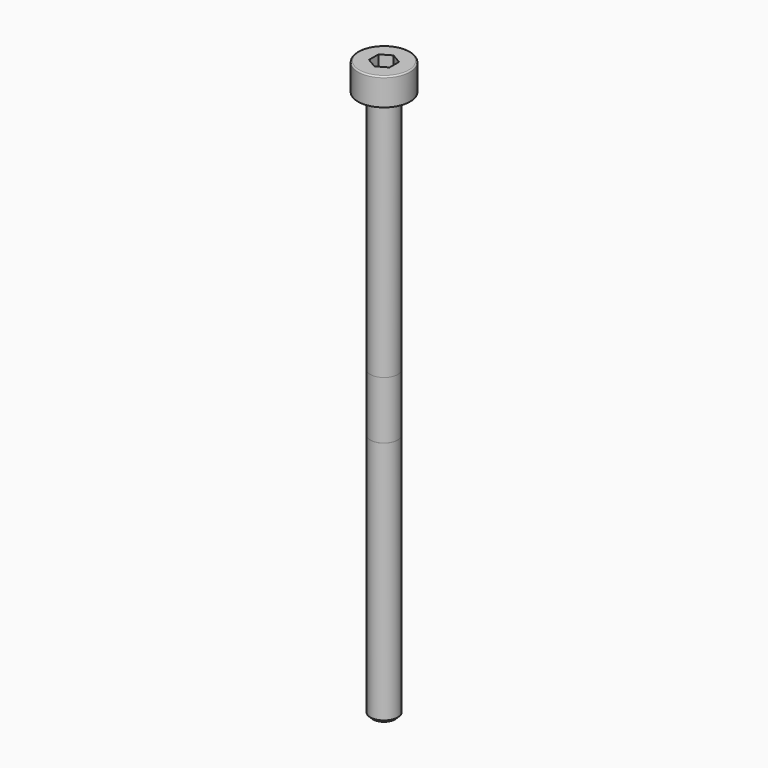
from build123d import *

# Parameters (mm, degrees)
F4_DEPTH = 1


with BuildPart() as f2:
    # F1 (on Front) → F2 (revolve)
    with BuildSketch(Plane.XZ):
        with BuildLine():
            Line((1.8, 2), (0, 2))
            Line((0, 2), (0, 0))
            Line((0, 0), (1.9, 0))
            Line((1.9, 0), (1.9, 1.9))
            ThreePointArc((1.9, 1.9), (1.8707106781, 1.9707106781), (1.8, 2))
        make_face()
    revolve(axis=Axis((0, 0, 1), (0, 0, 1)))

    # F3 (on face) → F4 (cut)
    with BuildSketch(Plane.XY.offset(2)):
        Polygon((0.75, -0.4330127019), (0.75, 0.4330127019), (0, 0.8660254038), (-0.75, 0.4330127019), (-0.75, -0.4330127019), (0, -0.8660254038), align=None)
    extrude(amount=-F4_DEPTH, mode=Mode.SUBTRACT)


with BuildPart() as f5_1:
    # F5: copy of F2
    add(f2.part)

    # F6 (on Front) → F7 (revolve)
    with BuildSketch(Plane.XZ):
        Polygon((1, 0), (0, 0), (0, -8), (0.8, -8), (1, -7.8), align=None)
    revolve(axis=Axis((0, 0, -4), (0, 0, -1)))


with BuildPart() as f8_1:
    # F8: copy of F2
    add(f2.part)

    # F9 (on Front) → F10 (revolve)
    with BuildSketch(Plane.XZ):
        Polygon((1, 0), (0, 0), (0, -10), (0.8, -10), (1, -9.8), align=None)
    revolve(axis=Axis((0, 0, -5), (0, 0, -1)))


with BuildPart() as f11_1:
    # F11: copy of F2
    add(f2.part)

    # F12 (on Front) → F13 (revolve)
    with BuildSketch(Plane.XZ):
        Polygon((1, 0), (0, 0), (0, -30), (0.8, -30), (1, -29.8), align=None)
    revolve(axis=Axis((0, 0, -15), (0, 0, -1)))


with BuildPart() as f14_1:
    # F14: copy of F2
    add(f2.part)

    # F15 (on Front) → F16 (revolve)
    with BuildSketch(Plane.XZ):
        Polygon((1, 0), (0, 0), (0, -40), (0.8, -40), (1, -39.8), (1, -22.0115470054), (0.98, -22), (1, -22), align=None)
    revolve(axis=Axis((0, 0, -20), (0, 0, -1)))


with BuildPart() as f17_1:
    # F17: copy of F2
    add(f2.part)

    # F18 (on Front) → F19 (revolve)
    with BuildSketch(Plane.XZ):
        Polygon((1, 0), (0, 0), (0, -6), (0.8, -6), (1, -5.8), align=None)
    revolve(axis=Axis((0, 0, -3), (0, 0, -1)))


with BuildPart() as f20_1:
    # F20: copy of F2
    add(f2.part)

    # F21 (on Front) → F22 (revolve)
    with BuildSketch(Plane.XZ):
        Polygon((1, 0), (0, 0), (0, -16), (0.8, -16), (1, -15.8), align=None)
    revolve(axis=Axis((0, 0, -8), (0, 0, 1)))


with BuildPart() as f23_1:
    # F23: copy of F2
    add(f2.part)

    # F24 (on Front) → F25 (revolve)
    with BuildSketch(Plane.XZ):
        Polygon((1, 0), (0, 0), (0, -12), (0.8, -12), (1, -11.8), align=None)
    revolve(axis=Axis((0, 0, -6), (0, 0, 1)))


with BuildPart() as f26_1:
    # F26: copy of F2
    add(f2.part)

    # F27 (on Front) → F28 (revolve)
    with BuildSketch(Plane.XZ):
        Polygon((1, 0), (0, 0), (0, -18), (0.8, -18), (1, -17.8), align=None)
    revolve(axis=Axis((0, 0, -9), (0, 0, 1)))


solid = Compound([f2.part, f5_1.part, f8_1.part, f11_1.part, f14_1.part, f17_1.part, f20_1.part, f23_1.part, f26_1.part])
